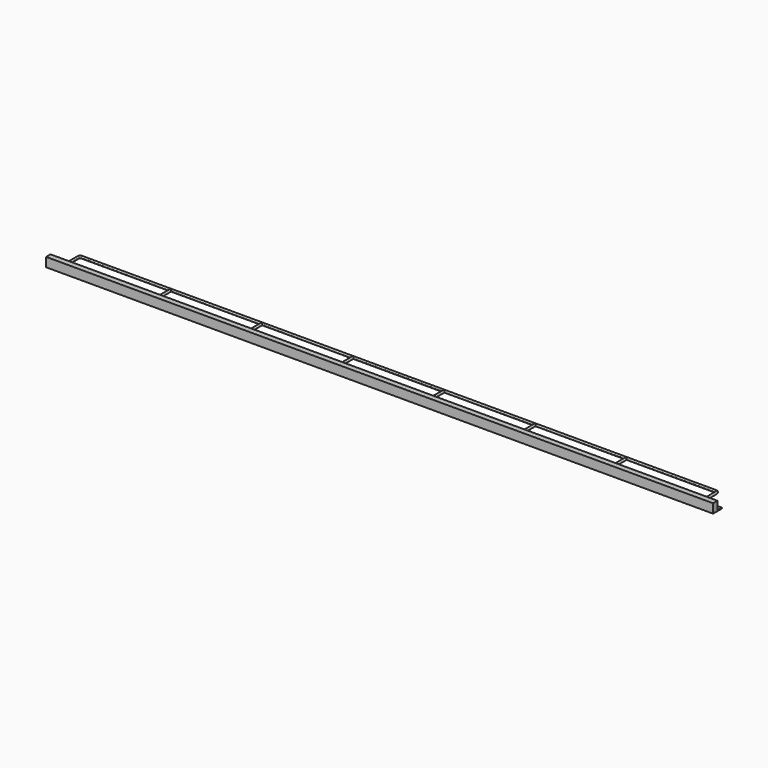
from build123d import *

# Parameters (mm, degrees)
F0_W          = 3635
F0_H          = 50
F1_DEPTH      = 15
F1_DEPTH_BACK = 15
F2_W          = 60
F2_H          = 30
F3_DEPTH      = 5
F4_W          = 60
F4_H          = 30
F4_H_2        = 15
F5_DEPTH      = 5
F6_R          = 6
F7_DEPTH      = 5
F9_DEPTH      = 5
F10_DEPTH     = 5
F11_DEPTH     = 5


# Not quite as in the source:
# - a feature names something its author has since deleted; it is built from what else it names


with BuildPart() as f1:
    # F0 (on Front) → F1 (new body, two sides)
    with BuildSketch(Plane.XZ) as f1_sk:
        Rectangle(F0_W, F0_H)
    extrude(amount=F1_DEPTH)
    extrude(f1_sk.sketch, amount=-F1_DEPTH_BACK)

    # F2 (on face) → F3 (join)
    with BuildSketch(Plane(origin=(0, 0, -25), x_dir=(1, 0, 0), z_dir=(0, 0, -1))):
        with Locations((-1787.5, -30)):
            Rectangle(F2_W, F2_H)
        Polygon((-1757.5, 15), (-1817.5, 15), (-1817.5, 0), (-1817.5, -15), (-1757.5, -15), align=None)
    extrude(amount=F3_DEPTH)

    # F4 (on face) → F5 (join)
    with BuildSketch(Plane(origin=(0, 0, -25), x_dir=(1, 0, 0), z_dir=(0, 0, -1))):
        with Locations((1787.5, -30)):
            Rectangle(F4_W, F4_H)
        with Locations((1787.5, -7.5)):
            Rectangle(F4_W, F4_H_2)
        with Locations((1787.5, 7.5)):
            Rectangle(F4_W, F4_H_2)
    extrude(amount=F5_DEPTH)

    # F6 (on face) → F7 (cut, through all)
    with BuildSketch(Plane(origin=(0, 0, -30), x_dir=(1, 0, 0), z_dir=(0, 0, -1))):
        with Locations((1782.5, -30)):
            Circle(F6_R)
    extrude(amount=-F7_DEPTH, mode=Mode.SUBTRACT)

    # F8 (on face) → F9 (cut, through all)
    with BuildSketch(Plane(origin=(0, 0, -30), x_dir=(1, 0, 0), z_dir=(0, 0, -1))):
        with BuildLine():
            ThreePointArc((-1788.5, -30), (-1782.5, -36), (-1776.5, -30))
            ThreePointArc((-1776.5, -30), (-1782.5, -24), (-1788.5, -30))
        make_face()
    extrude(amount=-F9_DEPTH, mode=Mode.SUBTRACT)

    # F10 (add): faces of the model
    f10_faces = [f1.faces().sort_by_distance(p)[0] for p in [
        (1787.5, 44.3291796068, -25),
        (-1816.8291796068, 30, -25),
    ]]
    extrude(f10_faces, amount=F10_DEPTH)

    # F11 (cut): faces of the model
    f11_faces = [f1.faces().sort_by_distance(p)[0] for p in [
        (-1787.6621744947, 14.5134765159, -30),
        (1787.6621744947, 14.5134765159, -30),
    ]]
    extrude(f11_faces, amount=-F11_DEPTH, mode=Mode.SUBTRACT)

    # F14: sweep along a path in F13
    with BuildLine(Plane.XY) as f14_path:
        Line((1737.5, 15), (1737.5, 105))
        ThreePointArc((1737.5, 105), (1734.5710678119, 112.0710678119), (1727.5, 115))
        Line((1727.5, 115), (-1727.5, 115))
        ThreePointArc((-1727.5, 115), (-1734.5710678119, 112.0710678119), (-1737.5, 105))
        Line((-1737.5, 105), (-1737.5, 15))
    # F12 (on face) → F14 (sweep)
    with BuildSketch(Plane(origin=(0, 15, 0), x_dir=(-1, 0, 0), z_dir=(0, 1, 0))):
        with BuildLine():
            ThreePointArc((-1731.5, 0), (-1741.7426406871, 4.2426406871), (-1737.5, -6))
            Line((-1737.5, -6), (-1737.5, 0))
            Line((-1737.5, 0), (-1731.5, 0))
        make_face()
        with BuildLine():
            Line((-1737.5, 0), (-1737.5, -6))
            ThreePointArc((-1737.5, -6), (-1733.2573593129, -4.2426406871), (-1731.5, 0))
            Line((-1731.5, 0), (-1737.5, 0))
        make_face()
    sweep(path=f14_path.line)

    # F15: sweep along a path in F13
    with BuildLine(Plane.XY) as f15_path:
        Line((-1241.0714285714, 115), (-1241.0714285714, 15))
    # F12 (on face) → F15 (sweep)
    with BuildSketch(Plane(origin=(0, 15, 0), x_dir=(-1, 0, 0), z_dir=(0, 1, 0))):
        with BuildLine():
            ThreePointArc((1247.0714285714, 0), (1241.0714285714, 6), (1235.0714285714, 0))
            Line((1235.0714285714, 0), (1241.0714285714, 0))
            Line((1241.0714285714, 0), (1247.0714285714, 0))
        make_face()
        with BuildLine():
            Line((1241.0714285714, 0), (1235.0714285714, 0))
            ThreePointArc((1235.0714285714, 0), (1241.0714285714, -6), (1247.0714285714, 0))
            Line((1247.0714285714, 0), (1241.0714285714, 0))
        make_face()
    sweep(path=f15_path.line)

    # F16: sweep along a path in F13
    with BuildLine(Plane.XY) as f16_path:
        Line((-744.6428571429, 115), (-744.6428571429, 15))
    # F12 (on face) → F16 (sweep)
    with BuildSketch(Plane(origin=(0, 15, 0), x_dir=(-1, 0, 0), z_dir=(0, 1, 0))):
        with BuildLine():
            ThreePointArc((750.6428571429, 0), (744.6428571429, 6), (738.6428571429, 0))
            Line((738.6428571429, 0), (744.6428571429, 0))
            Line((744.6428571429, 0), (750.6428571429, 0))
        make_face()
        with BuildLine():
            Line((744.6428571429, 0), (738.6428571429, 0))
            ThreePointArc((738.6428571429, 0), (744.6428571429, -6), (750.6428571429, 0))
            Line((750.6428571429, 0), (744.6428571429, 0))
        make_face()
    sweep(path=f16_path.line)

    # F17: sweep along a path in F13
    with BuildLine(Plane.XY) as f17_path:
        Line((-248.2142857143, 115), (-248.2142857143, 15))
    # F12 (on face) → F17 (sweep)
    with BuildSketch(Plane(origin=(0, 15, 0), x_dir=(-1, 0, 0), z_dir=(0, 1, 0))):
        with BuildLine():
            ThreePointArc((254.2142857143, 0), (248.2142857143, 6), (242.2142857143, 0))
            Line((242.2142857143, 0), (248.2142857143, 0))
            Line((248.2142857143, 0), (254.2142857143, 0))
        make_face()
        with BuildLine():
            Line((248.2142857143, 0), (242.2142857143, 0))
            ThreePointArc((242.2142857143, 0), (248.2142857143, -6), (254.2142857143, 0))
            Line((254.2142857143, 0), (248.2142857143, 0))
        make_face()
    sweep(path=f17_path.line)

    # F18: sweep along a path in F13
    with BuildLine(Plane.XY) as f18_path:
        Line((248.2142857143, 15), (248.2142857143, 115))
    # F12 (on face) → F18 (sweep)
    with BuildSketch(Plane(origin=(0, 15, 0), x_dir=(-1, 0, 0), z_dir=(0, 1, 0))):
        with BuildLine():
            ThreePointArc((-242.2142857143, 0), (-248.2142857143, 6), (-254.2142857143, 0))
            Line((-254.2142857143, 0), (-248.2142857143, 0))
            Line((-248.2142857143, 0), (-242.2142857143, 0))
        make_face()
        with BuildLine():
            Line((-248.2142857143, 0), (-254.2142857143, 0))
            ThreePointArc((-254.2142857143, 0), (-248.2142857143, -6), (-242.2142857143, 0))
            Line((-242.2142857143, 0), (-248.2142857143, 0))
        make_face()
    sweep(path=f18_path.line)

    # F19: sweep along a path in F13
    with BuildLine(Plane.XY) as f19_path:
        Line((744.6428571429, 15), (744.6428571429, 115))
    # F12 (on face) → F19 (sweep)
    with BuildSketch(Plane(origin=(0, 15, 0), x_dir=(-1, 0, 0), z_dir=(0, 1, 0))):
        with BuildLine():
            ThreePointArc((-738.6428571429, 0), (-744.6428571429, 6), (-750.6428571429, 0))
            Line((-750.6428571429, 0), (-744.6428571429, 0))
            Line((-744.6428571429, 0), (-738.6428571429, 0))
        make_face()
        with BuildLine():
            Line((-744.6428571429, 0), (-750.6428571429, 0))
            ThreePointArc((-750.6428571429, 0), (-744.6428571429, -6), (-738.6428571429, 0))
            Line((-738.6428571429, 0), (-744.6428571429, 0))
        make_face()
    sweep(path=f19_path.line)

    # F20: sweep along a path in F13
    with BuildLine(Plane.XY) as f20_path:
        Line((1241.0714285714, 15), (1241.0714285714, 115))
    # F12 (on face) → F20 (sweep)
    with BuildSketch(Plane(origin=(0, 15, 0), x_dir=(-1, 0, 0), z_dir=(0, 1, 0))):
        with BuildLine():
            ThreePointArc((-1235.0714285714, 0), (-1241.0714285714, 6), (-1247.0714285714, 0))
            Line((-1247.0714285714, 0), (-1241.0714285714, 0))
            Line((-1241.0714285714, 0), (-1235.0714285714, 0))
        make_face()
        with BuildLine():
            Line((-1241.0714285714, 0), (-1247.0714285714, 0))
            ThreePointArc((-1247.0714285714, 0), (-1241.0714285714, -6), (-1235.0714285714, 0))
            Line((-1235.0714285714, 0), (-1241.0714285714, 0))
        make_face()
    sweep(path=f20_path.line)


solid = f1.part
